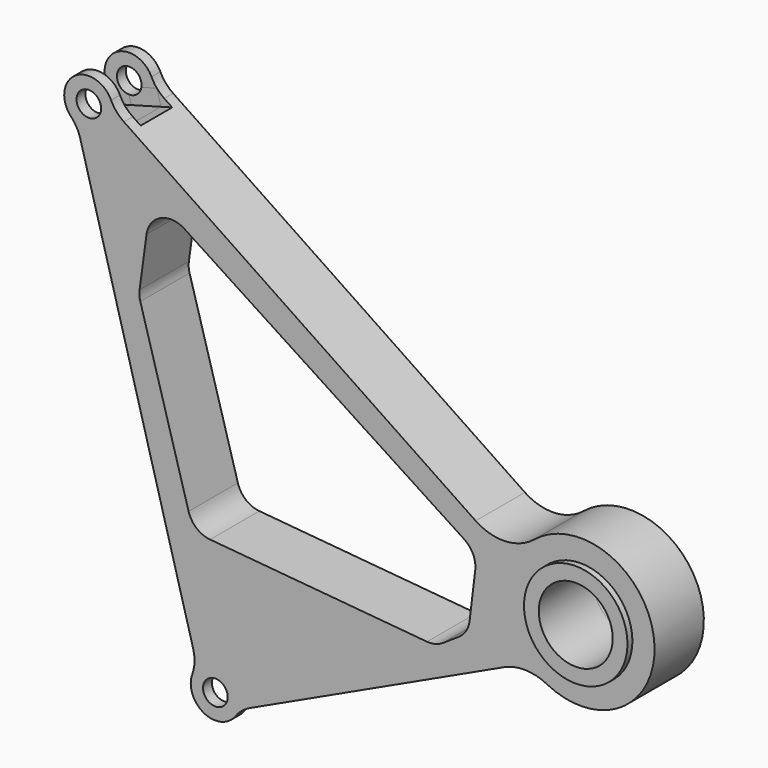
from build123d import *

# Parameters (mm, degrees)
F0_R           = 10
F0_R_2         = 30
F1_DEPTH       = 50
F3_W           = 32
F3_H           = 46.9773098714
F4_DEPTH       = 36
F4_DEPTH_BACK  = 36
F7_W           = 64.344675952
F7_H           = 32
F8_DEPTH       = 35
F8_DEPTH_BACK  = 25
F10_DEPTH      = 100
F11_R          = 20
F12_R          = 42
F12_R_2        = 30
F13_DEPTH      = 5
F14_R          = 42
F14_R_2        = 30
F15_DEPTH      = 5
F16_W          = 32
F16_H          = 12.6297663026
F17_DEPTH      = 25
F17_DEPTH_BACK = 25


# Not quite as in the source:
# - a feature names something its author has since deleted; it is built from what else it names


with BuildPart() as f1:
    # F0 (on Front) → F1 (new body)
    with BuildSketch(Plane.XZ):
        with BuildLine():
            ThreePointArc((-62.5780437897, -52.7205259787), (-44.9107725801, -48.9739327439), (-27.3963571385, -53.3801425208))
            ThreePointArc((-27.3963571385, -53.3801425208), (59.6815194776, 6.173834533), (-37.7432491465, 46.6416889045))
            ThreePointArc((-37.7432491465, 46.6416889045), (-61.1526251037, 37.7745700431), (-85.2484645361, 44.5580206149))
            Line((-85.2484645361, 44.5580206149), (-370.7956962097, 236.8532567171))
            ThreePointArc((-370.7956962097, 236.8532567171), (-376.7925336048, 242.1856420807), (-381.1612781983, 248.9169467897))
            ThreePointArc((-381.1612781983, 248.9169467897), (-410.6071858154, 256.8281563435), (-413.6417851947, 226.4894035906))
            ThreePointArc((-413.6417851947, 226.4894035906), (-409.1637807856, 220.5019975774), (-406.3054242786, 213.5932095263))
            Line((-406.3054242786, 213.5932095263), (-314.4991596079, -121.5832610972))
            ThreePointArc((-314.4991596079, -121.5832610972), (-313.4615655347, -130.8078667851), (-315.293607643, -139.9080631166))
            ThreePointArc((-315.293607643, -139.9080631166), (-305.9378740774, -164.4922463623), (-280.3150583777, -158.5438741459))
            ThreePointArc((-280.3150583777, -158.5438741459), (-275.1112486364, -152.9838392789), (-268.6751253171, -148.913220141))
            Line((-268.6751253171, -148.913220141), (-62.5780437897, -52.7205259787))
        make_face()
        with Locations((-296.5337380309, -146.8411210378)):
            Circle(F0_R, mode=Mode.SUBTRACT)
        Circle(F0_R_2, mode=Mode.SUBTRACT)
        with Locations((-399.2431908367, 240.3703430585)):
            Circle(F0_R, mode=Mode.SUBTRACT)
    extrude(amount=F1_DEPTH)

    # F3 (on face) → F4 (cut, two sides)
    with BuildSketch(Plane(origin=(-323.5290376394, 0, -88.6159831057), x_dir=(0, -1, 0), z_dir=(-0.9644750818, 0, -0.2641738379))) as f4_sk:
        with Locations((25, 344.0173126814)):
            Rectangle(F3_W, F3_H)
    extrude(amount=F4_DEPTH, mode=Mode.SUBTRACT)
    extrude(f4_sk.sketch, amount=-F4_DEPTH_BACK, mode=Mode.SUBTRACT)

    # F7 (on offset) → F8 (cut, two sides)
    with BuildSketch(Plane(origin=(9.0113675019, 0, -19.3072515422), x_dir=(0.9061594556, 0, 0.422936214), z_dir=(0.422936214, 0, -0.9061594556))) as f8_sk:
        with Locations((-346.1694030438, 25)):
            Rectangle(F7_W, F7_H)
    extrude(amount=-F8_DEPTH, mode=Mode.SUBTRACT)
    extrude(f8_sk.sketch, amount=F8_DEPTH_BACK, mode=Mode.SUBTRACT)

    # F9 (on face) → F10 (cut)
    with BuildSketch(Plane.XZ.offset(50)):
        Polygon((-348.2052087784, 193.6148256063), (-358.6101531982, 116.7783439159), (-314.4991596079, -37.6950278878), (-117.6957413554, -55.3033873439), (-91.2832021713, -37.6950278878), (-84.079772234, 21.5331036597), align=None)
    extrude(amount=-F10_DEPTH, mode=Mode.SUBTRACT)

    # F11
    f11_edges = [f1.edges().sort_by_distance(p)[0] for p in [
        (-348.205209, -25, 193.614826),
        (-358.610153, -25, 116.778344),
        (-84.079772, -25, 21.533104),
        (-91.283202, -25, -37.695028),
        (-117.695741, -25, -55.303387),
        (-314.49916, -25, -37.695028),
    ]]
    fillet(f11_edges, radius=F11_R)

    # F12 (on face) → F13 (join)
    with BuildSketch(Plane.XZ.offset(50)):
        Circle(F12_R)
        Circle(F12_R_2, mode=Mode.SUBTRACT)
    extrude(amount=F13_DEPTH)

    # F14 (on face) → F15 (join)
    with BuildSketch(Plane(origin=(0, 0, 0), x_dir=(-1, 0, 0), z_dir=(0, 1, 0))):
        Circle(F14_R)
        Circle(F14_R_2, mode=Mode.SUBTRACT)
    extrude(amount=F15_DEPTH)

    # F16 (on face) → F17 (cut, two sides)
    with BuildSketch(Plane(origin=(-288.8079346956, 0, -79.1057249405), x_dir=(0, -1, 0), z_dir=(-0.9644750818, 0, -0.2641738379))) as f17_sk:
        with Locations((25, 326.843540897)):
            Rectangle(F16_W, F16_H)
    extrude(amount=F17_DEPTH, mode=Mode.SUBTRACT)
    extrude(f17_sk.sketch, amount=-F17_DEPTH_BACK, mode=Mode.SUBTRACT)


solid = f1.part
